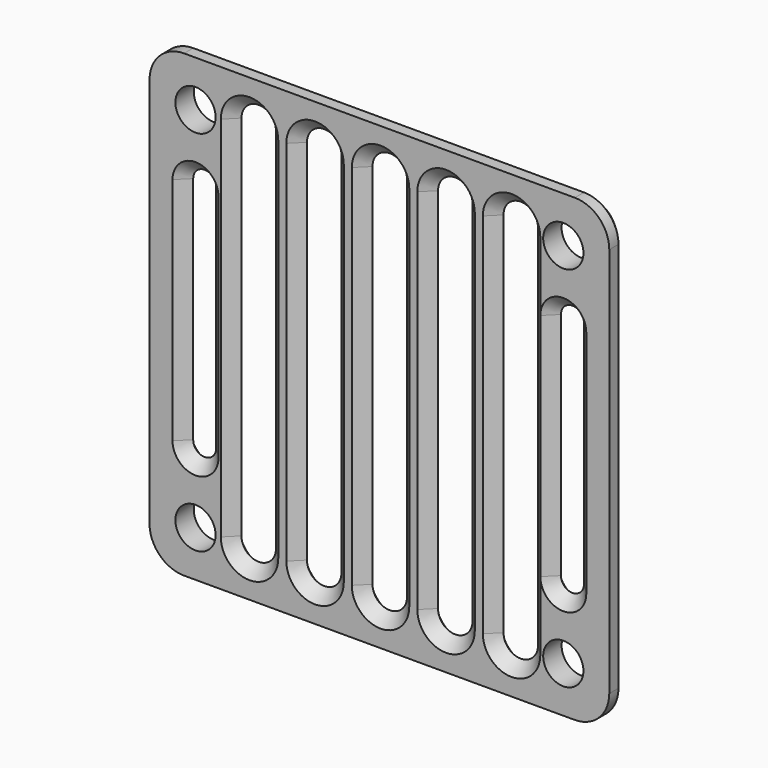
from build123d import *

# Parameters (mm, degrees)
F0_R     = 1.75
F1_DEPTH = 2
F2_SIZE  = 0.99999


# Not quite as in the source:
# - a fillet or chamfer is up to 0.001 mm smaller than in the source, because OpenCascade refuses the exact size


with BuildPart() as f1:
    # F0 (on Front) → F1 (new body)
    with BuildSketch(Plane.XZ):
        with BuildLine():
            ThreePointArc((20, 17), (19.1213203436, 19.1213203436), (17, 20))
            Line((17, 20), (-17, 20))
            ThreePointArc((-17, 20), (-19.1213203436, 19.1213203436), (-20, 17))
            Line((-20, 17), (-20, -17))
            ThreePointArc((-20, -17), (-19.1213203436, -19.1213203436), (-17, -20))
            Line((-17, -20), (17, -20))
            ThreePointArc((17, -20), (19.1213203436, -19.1213203436), (20, -17))
            Line((20, -17), (20, 17))
        make_face()
        with Locations((-16, -16)):
            Circle(F0_R, mode=Mode.SUBTRACT)
        with Locations((16, -16)):
            Circle(F0_R, mode=Mode.SUBTRACT)
        with BuildLine():
            ThreePointArc((-17, 10), (-16, 11), (-15, 10))
            Line((-15, 10), (-15, -10))
            ThreePointArc((-15, -10), (-16, -11), (-17, -10))
            Line((-17, -10), (-17, 10))
        make_face(mode=Mode.SUBTRACT)
        with BuildLine():
            ThreePointArc((-9.8, -16), (-11.3, -17.5), (-12.8, -16))
            Line((-12.8, -16), (-12.8, 16))
            ThreePointArc((-12.8, 16), (-11.3, 17.5), (-9.8, 16))
            Line((-9.8, 16), (-9.8, -16))
        make_face(mode=Mode.SUBTRACT)
        with BuildLine():
            ThreePointArc((-4.1, -16), (-5.6, -17.5), (-7.1, -16))
            Line((-7.1, -16), (-7.1, 16))
            ThreePointArc((-7.1, 16), (-5.6, 17.5), (-4.1, 16))
            Line((-4.1, 16), (-4.1, -16))
        make_face(mode=Mode.SUBTRACT)
        with Locations((-16, 16)):
            Circle(F0_R, mode=Mode.SUBTRACT)
        with BuildLine():
            ThreePointArc((1.6, -16), (0.1, -17.5), (-1.4, -16))
            Line((-1.4, -16), (-1.4, 16))
            ThreePointArc((-1.4, 16), (0.1, 17.5), (1.6, 16))
            Line((1.6, 16), (1.6, -16))
        make_face(mode=Mode.SUBTRACT)
        with BuildLine():
            ThreePointArc((7.3, -16), (5.8, -17.5), (4.3, -16))
            Line((4.3, -16), (4.3, 16))
            ThreePointArc((4.3, 16), (5.8, 17.5), (7.3, 16))
            Line((7.3, 16), (7.3, -16))
        make_face(mode=Mode.SUBTRACT)
        with BuildLine():
            ThreePointArc((10, 16), (11.5, 17.5), (13, 16))
            Line((13, 16), (13, -16))
            ThreePointArc((13, -16), (11.5, -17.5), (10, -16))
            Line((10, -16), (10, 16))
        make_face(mode=Mode.SUBTRACT)
        with BuildLine():
            Line((15, -10), (15, 10))
            ThreePointArc((15, 10), (16, 11), (17, 10))
            Line((17, 10), (17, -10))
            ThreePointArc((17, -10), (16, -11), (15, -10))
        make_face(mode=Mode.SUBTRACT)
        with Locations((16, 16)):
            Circle(F0_R, mode=Mode.SUBTRACT)
    extrude(amount=F1_DEPTH)

    # F2 (size 1 in the source; OpenCascade refuses exactly that, so slightly less here)
    f2_edges = [f1.edges().sort_by_distance(p)[0] for p in [
        (17, 0, 0),
        (15, 0, 0),
        (16, 0, 11),
        (16, 0, -11),
        (13, 0, 0),
        (7.3, 0, 0),
        (1.6, 0, 0),
        (-4.1, 0, 0),
        (-9.8, 0, 0),
        (-15, 0, 0),
        (-9.8, -2, 0),
        (-15, -2, 0),
        (-4.1, -2, 0),
        (1.6, -2, 0),
        (7.3, -2, 0),
        (13, -2, 0),
        (17, -2, 0),
        (-20, 0, 0),
    ]]
    chamfer(f2_edges, length=F2_SIZE)


solid = f1.part
